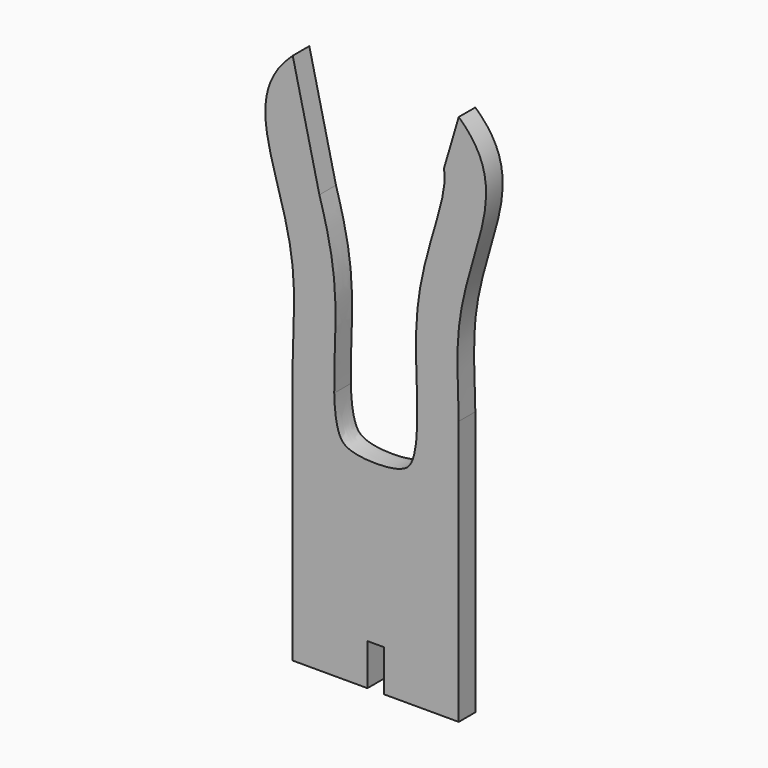
from build123d import *

# Parameters (mm, degrees)
F1_DEPTH = 25.4


# Not quite as in the source:
# - ends of sketch curves that miss each other by under 0.0002 mm in the source are joined
# - the dataset's text gives a spline's control points without its knots; the knots are read off the source's solid


with BuildPart() as f1:
    # F0 (on Front) → F1 (new body)
    with BuildSketch(Plane.XZ):
        with BuildLine():
            Line((50.7886661445, -169.501300597), (101.6, -169.501300597))
            Line((101.6, -169.501300597), (101.6, -150.3751168758))
            add(Edge.make_bspline(
                [(101.6, -150.3751168758), (101.0803773196, -117.7440464819), (98.4617716942, -82.917940171), (101.6, -51.0090794925)],
                knots=[0.348093007, 0.348093007, 0.348093007, 0.348093007, 0.5112644576, 0.5112644576, 0.5112644576, 0.5112644576], degree=3))
            Line((101.6, -51.0090794925), (101.6, 177.5909205075))
            Line((101.6, 177.5909205075), (83.4101587534, 115.8730164172))
            add(Edge.make_bspline(
                [(50.7886661445, -169.501300597), (50.9026473085, -164.4666491573), (50.9162725112, -153.6138316114), (50.4636858885, -135.7972792214), (49.8021912395, -116.5746729514), (49.3576545415, -99.7826123267), (49.2531559515, -85.9749958934), (49.335688401, -77.2034653803), (49.5179812371, -70.1086042792), (49.7202521595, -64.7501100209), (49.9956887424, -59.3560667778), (50.3524545586, -53.9266908033), (50.7241762184, -49.3775107215), (51.0715100868, -45.715899498), (51.4506198285, -42.0687688389), (51.9791682398, -37.5633415444), (52.9337939166, -30.4589860124), (54.3142565918, -21.7807556023), (56.2181350891, -11.6920282806), (58.3180902632, -1.9300834326), (60.5643464457, 7.5051162117), (62.9086527251, 16.6139933437), (66.1031990118, 28.3243025883), (70.1123580141, 42.1464064382), (74.6114430285, 57.4069567688), (78.4965590416, 71.284335377), (81.5155021001, 83.6774933313), (83.1641645829, 92.6506749789), (83.9402132699, 98.9504509527), (84.2613379993, 103.228677272), (84.3389906187, 107.0641497537), (84.19830623, 110.479260656), (83.8806341112, 113.3848479047), (83.5738558843, 115.1024571447), (83.4101587534, 115.8730164172)],
                knots=[0.3137294715, 0.3137294715, 0.3137294715, 0.3137294715, 0.34375, 0.375, 0.40625, 0.4375, 0.453125, 0.46875, 0.4765625, 0.484375, 0.4921875, 0.5, 0.5078125, 0.51171875, 0.515625, 0.5234375, 0.53125, 0.546875, 0.5625, 0.578125, 0.59375, 0.609375, 0.625, 0.65625, 0.6875, 0.71875, 0.75, 0.78125, 0.796875, 0.8125, 0.828125, 0.84375, 0.859375, 0.8729112364, 0.8729112364, 0.8729112364, 0.8729112364], degree=3))
        make_face()
        Polygon((0, -279.6090794925), (-101.6, -279.6090794925), (-101.6, -474.301300597), (-10.16, -474.301300597), (-10.16, -423.501300597), (10.16, -423.501300597), (10.16, -474.301300597), (101.6, -474.301300597), (101.6, -279.6090794925), align=None)
        with BuildLine():
            add(Edge.make_bspline(
                [(0, -279.6090794925), (-85.4963409355, -279.6090794925), (-100.3950962884, -230.5628557419), (-101.6, -169.501300597)],
                knots=[0, 0, 0, 0, 0.3157141006, 0.3157141006, 0.3157141006, 0.3157141006], degree=3))
            Line((-101.6, -169.501300597), (-101.6, -279.6090794925))
            Line((-101.6, -279.6090794925), (0, -279.6090794925))
        make_face()
        with BuildLine():
            add(Edge.make_bspline(
                [(0, -279.6090794925), (85.4963409355, -279.6090794925), (100.3950962884, -230.5628557419), (101.6, -169.501300597)],
                knots=[0, 0, 0, 0, 0.3157141006, 0.3157141006, 0.3157141006, 0.3157141006], degree=3))
            Line((0, -279.6090794925), (101.6, -279.6090794925))
            Line((101.6, -279.6090794925), (101.6, -169.501300597))
        make_face()
        with BuildLine():
            Line((-50.7886661445, -169.501300597), (-101.6, -169.501300597))
            add(Edge.make_bspline(
                [(0, -279.6090794925), (-85.4963409355, -279.6090794925), (-100.3950962884, -230.5628557419), (-101.6, -169.501300597)],
                knots=[0, 0, 0, 0, 0.3157141006, 0.3157141006, 0.3157141006, 0.3157141006], degree=3))
            add(Edge.make_bspline(
                [(0, -279.6090794925), (85.4963409355, -279.6090794925), (100.3950962884, -230.5628557419), (101.6, -169.501300597)],
                knots=[0, 0, 0, 0, 0.3157141006, 0.3157141006, 0.3157141006, 0.3157141006], degree=3))
            Line((101.6, -169.501300597), (50.7886661445, -169.501300597))
            add(Edge.make_bspline(
                [(0, -228.8090831103), (3.269781633, -228.8090831103), (9.3419832707, -228.6229310101), (17.0615138024, -227.8828258437), (23.423495404, -226.7969938358), (28.4909159521, -225.4945264796), (32.3736912078, -224.1069579249), (35.2400479212, -222.7466575878), (37.3149032346, -221.4771956614), (38.8571376876, -220.2857794099), (40.1171978502, -219.0737094322), (41.2909312987, -217.6756427871), (42.4914822353, -215.9017000487), (43.7502167423, -213.5822216388), (45.0397816284, -210.5965677874), (46.3038548634, -206.8807266614), (47.4808945474, -202.4195546791), (48.8664504568, -195.5047850788), (50.1551603902, -185.1503489807), (50.6559263277, -175.1419911871), (50.7839981189, -169.707491524), (50.7886661445, -169.501300597)],
                knots=[0, 0, 0, 0, 0.015625, 0.03125, 0.046875, 0.0625, 0.078125, 0.09375, 0.109375, 0.125, 0.140625, 0.15625, 0.171875, 0.1875, 0.203125, 0.21875, 0.234375, 0.25, 0.28125, 0.3125, 0.3137294715, 0.3137294715, 0.3137294715, 0.3137294715], degree=3))
            add(Edge.make_bspline(
                [(0, -228.8090831103), (-3.269781633, -228.8090831103), (-9.3419832707, -228.6229310101), (-17.0615138024, -227.8828258437), (-23.423495404, -226.7969938358), (-28.4909159521, -225.4945264796), (-32.3736912078, -224.1069579249), (-35.2400479212, -222.7466575878), (-37.3149032346, -221.4771956614), (-38.8571376876, -220.2857794099), (-40.1171978502, -219.0737094322), (-41.2909312987, -217.6756427871), (-42.4914822353, -215.9017000487), (-43.7502167423, -213.5822216388), (-45.0397816284, -210.5965677874), (-46.3038548634, -206.8807266614), (-47.4808945474, -202.4195546791), (-48.8664504568, -195.5047850788), (-50.1551603902, -185.1503489807), (-50.6559263277, -175.1419911871), (-50.7839981189, -169.707491524), (-50.7886661445, -169.501300597)],
                knots=[0, 0, 0, 0, 0.015625, 0.03125, 0.046875, 0.0625, 0.078125, 0.09375, 0.109375, 0.125, 0.140625, 0.15625, 0.171875, 0.1875, 0.203125, 0.21875, 0.234375, 0.25, 0.28125, 0.3125, 0.3137294715, 0.3137294715, 0.3137294715, 0.3137294715], degree=3))
        make_face()
        with BuildLine():
            Line((-101.6, -150.3751168758), (-101.6, -169.501300597))
            Line((-101.6, -169.501300597), (-50.7886661445, -169.501300597))
            add(Edge.make_bspline(
                [(-50.7886661445, -169.501300597), (-50.9026473085, -164.4666491573), (-50.9162725112, -153.6138316114), (-50.4636858885, -135.7972792214), (-49.8021912395, -116.5746729514), (-49.3576545415, -99.7826123267), (-49.2531559515, -85.9749958934), (-49.335688401, -77.2034653803), (-49.5179812371, -70.1086042792), (-49.7202521595, -64.7501100209), (-49.9956887424, -59.3560667778), (-50.3524545586, -53.9266908033), (-50.7241762184, -49.3775107215), (-51.0715100868, -45.715899498), (-51.4506198285, -42.0687688389), (-51.9791682398, -37.5633415444), (-52.9337939166, -30.4589860124), (-54.3142565918, -21.7807556023), (-56.2181350891, -11.6920282806), (-58.3180902632, -1.9300834326), (-60.5643464457, 7.5051162117), (-62.9086527251, 16.6139933437), (-65.7384121018, 26.9870962556), (-67.776423883, 34.0808531414), (-68.9897870959, 38.254237712)],
                knots=[0.3137294715, 0.3137294715, 0.3137294715, 0.3137294715, 0.34375, 0.375, 0.40625, 0.4375, 0.453125, 0.46875, 0.4765625, 0.484375, 0.4921875, 0.5, 0.5078125, 0.51171875, 0.515625, 0.5234375, 0.53125, 0.546875, 0.5625, 0.578125, 0.59375, 0.609375, 0.625, 0.6491130923, 0.6491130923, 0.6491130923, 0.6491130923], degree=3))
            Line((-68.9897870959, 38.254237712), (-101.6, 177.5909205075))
            Line((-101.6, 177.5909205075), (-101.6, -51.0090794925))
            add(Edge.make_bspline(
                [(-101.6, -150.3751168758), (-101.0803773196, -117.7440464819), (-98.4617716942, -82.917940171), (-101.6, -51.0090794925)],
                knots=[0.348093007, 0.348093007, 0.348093007, 0.348093007, 0.5112644576, 0.5112644576, 0.5112644576, 0.5112644576], degree=3))
        make_face()
        with BuildLine():
            Line((101.6, 177.5909205075), (101.6, -51.0090794925))
            add(Edge.make_bspline(
                [(101.6, -51.0090794925), (110.9997063058, 44.5652030968), (172.0461866031, 113.9677517687), (101.6, 177.5909205075)],
                knots=[0.5112644576, 0.5112644576, 0.5112644576, 0.5112644576, 1, 1, 1, 1], degree=3))
        make_face()
        with BuildLine():
            add(Edge.make_bspline(
                [(-101.6, -51.0090794925), (-110.9997063058, 44.5652030968), (-172.0461866031, 113.9677517687), (-101.6, 177.5909205075)],
                knots=[0.5112644576, 0.5112644576, 0.5112644576, 0.5112644576, 1, 1, 1, 1], degree=3))
            Line((-101.6, -51.0090794925), (-101.6, 177.5909205075))
        make_face()
    extrude(amount=F1_DEPTH)


solid = f1.part
